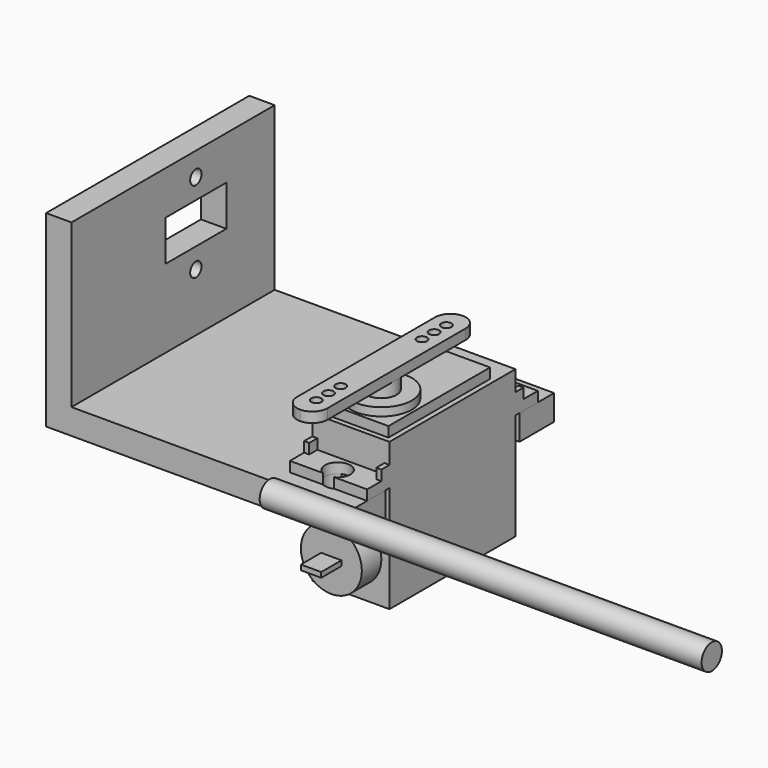
from build123d import *

# Parameters (mm, degrees)
F0_W      = 15.2
F0_H      = 31
F1_DEPTH  = 21
F3_DEPTH  = 2
F5_DEPTH  = 14.4
F4_W      = 1
F4_H      = 2
F6_DEPTH  = 2
F7_DEPTH  = 6
F8_R      = 6
F9_DEPTH  = 3.6
F8_W      = 13.2
F8_H      = 25
F10_DEPTH = 2
F11_R     = 3
F12_DEPTH = 2.6
F13_R     = 6
F14_DEPTH = 4.8
F15_W     = 4
F15_H     = 1
F16_DEPTH = 5
F18_DEPTH = 2
F19_R     = 1
F20_DEPTH = 2
F22_DEPTH = 5
F23_W     = 5
F23_H     = 50
F24_DEPTH = 32
F25_R     = 1.4
F25_W     = 15
F25_H     = 8
F26_DEPTH = 5
F27_R     = 2.7
F28_DEPTH = 2
F29_R     = 2.5
F30_DEPTH = 87


# Not quite as in the source:
# - an extrude ends at something that could not be found from the text; its depth is read off the source's solid


with BuildPart() as f1:
    # F0 (on Top) → F1 (new body)
    with BuildSketch(Plane.XY):
        with Locations((-7.6, 15.5)):
            Rectangle(F0_W, F0_H)
    extrude(amount=F1_DEPTH)

    # F2 (on face) → F3 (join)
    with BuildSketch(Plane.XY.offset(21)):
        Polygon((0, 36.5), (-15.2, 36.5), (-15.2, 31), (-15.2, 0), (-15.2, -5.5), (0, -5.5), (0, 0), (0, 31), align=None)
    extrude(amount=F3_DEPTH)

    # F4 (on face) → F5 (cut, through all)
    with BuildSketch(Plane.XY.offset(23)):
        with BuildLine():
            ThreePointArc((-6.5102752641, 36.5), (-7.6, 36.75), (-8.6897247359, 36.5))
            Line((-8.6897247359, 36.5), (-6.5102752641, 36.5))
        make_face()
        with BuildLine():
            Line((-6.5102752641, 36.5), (-8.6897247359, 36.5))
            ThreePointArc((-8.6897247359, 36.5), (-8.9277213865, 32.1317091985), (-5.1, 34.25))
            ThreePointArc((-5.1, 34.25), (-5.4817091985, 35.5777213865), (-6.5102752641, 36.5))
        make_face()
        with BuildLine():
            Line((-6.5102752641, -5.5), (-8.6897247359, -5.5))
            ThreePointArc((-8.6897247359, -5.5), (-7.6, -5.75), (-6.5102752641, -5.5))
        make_face()
        with BuildLine():
            ThreePointArc((-5.1, -3.25), (-8.9277213865, -1.1317091985), (-8.6897247359, -5.5))
            Line((-8.6897247359, -5.5), (-6.5102752641, -5.5))
            ThreePointArc((-6.5102752641, -5.5), (-5.4817091985, -4.5777213865), (-5.1, -3.25))
        make_face()
    extrude(amount=-F5_DEPTH, mode=Mode.SUBTRACT)

    # F4 (on face) → F6 (join)
    with BuildSketch(Plane.XY.offset(23)):
        with Locations((-14.7, 32)):
            Rectangle(F4_W, F4_H)
        with Locations((-0.5, 32)):
            Rectangle(F4_W, F4_H)
        with Locations((-0.5, -1)):
            Rectangle(F4_W, F4_H)
        with Locations((-14.7, -1)):
            Rectangle(F4_W, F4_H)
    extrude(amount=F6_DEPTH)

    # F4 (on face) → F7 (join)
    with BuildSketch(Plane.XY.offset(23)):
        Polygon((-14.2, 31), (-15.2, 31), (-15.2, 0), (-14.2, 0), (-1, 0), (0, 0), (0, 31), (-1, 31), align=None)
    extrude(amount=F7_DEPTH)

    # F8 (on face) → F9 (join)
    with BuildSketch(Plane.XY.offset(29)):
        with Locations((-7.6, 7.5)):
            Circle(F8_R)
    extrude(amount=F9_DEPTH)

    # F8 (on face) → F10 (join)
    with BuildSketch(Plane.XY.offset(29)):
        with Locations((-7.6, 13.5)):
            Rectangle(F8_W, F8_H)
        with Locations((-7.6, 7.5)):
            Circle(F8_R, mode=Mode.SUBTRACT)
    extrude(amount=F10_DEPTH)

    # F13 (on face) → F14 (join)
    with BuildSketch(Plane.XZ):
        with Locations((-7.6, 8.1)):
            Circle(F13_R)
    extrude(amount=F14_DEPTH)

    # F15 (on face) → F16 (join)
    with BuildSketch(Plane.XZ.offset(4.8)):
        with Locations((-7.6, 8.1)):
            Rectangle(F15_W, F15_H)
    extrude(amount=F16_DEPTH)


with BuildPart() as f12:
    # F11 (on face) → F12 (new body)
    with BuildSketch(Plane.XY.offset(32.6)):
        with Locations((-7.6, 7.5)):
            Circle(F11_R)
    extrude(amount=F12_DEPTH)

    # F17 (on face) → F18 (join)
    with BuildSketch(Plane.XY.offset(35.2)):
        with BuildLine():
            ThreePointArc((-7.6, 27.5), (-9.7213203436, 26.6213203436), (-10.6, 24.5))
            Line((-10.6, 24.5), (-10.6, -9.5))
            ThreePointArc((-10.6, -9.5), (-9.7213203436, -11.6213203436), (-7.6, -12.5))
            ThreePointArc((-7.6, -12.5), (-5.4786796564, -11.6213203436), (-4.6, -9.5))
            Line((-4.6, -9.5), (-4.6, 24.5))
            ThreePointArc((-4.6, 24.5), (-5.4786796564, 26.6213203436), (-7.6, 27.5))
        make_face()
    extrude(amount=F18_DEPTH)

    # F19 (on face) → F20 (cut, through all)
    with BuildSketch(Plane.XY.offset(37.2)):
        with Locations((-7.6, 23.5)):
            Circle(F19_R)
        with Locations((-7.6, -8.5)):
            Circle(F19_R)
        with Locations((-7.6, 20.5)):
            Circle(F19_R)
        with Locations((-7.6, 17.5)):
            Circle(F19_R)
        with Locations((-7.6, -2.5)):
            Circle(F19_R)
        with Locations((-7.6, -5.5)):
            Circle(F19_R)
    extrude(amount=-F20_DEPTH, mode=Mode.SUBTRACT)


with BuildPart() as f22:
    # F21 (on face) → F22 (new body)
    with BuildSketch(Plane(origin=(0, 0, 21), x_dir=(1, 0, 0), z_dir=(0, 0, -1))):
        with BuildLine():
            Line((0, 5.5), (0, 9.5))
            Line((0, 9.5), (-60, 9.5))
            Line((-60, 9.5), (-60, -40.5))
            Line((-60, -40.5), (0, -40.5))
            Line((0, -40.5), (0, -32))
            Line((0, -32), (-6.5102752641, -32))
            ThreePointArc((-6.5102752641, -32), (-5.4817091985, -32.9222786135), (-5.1, -34.25))
            ThreePointArc((-5.1, -34.25), (-8.9277213865, -36.3682908015), (-8.6897247359, -32))
            Line((-8.6897247359, -32), (-16, -32))
            Line((-16, -32), (-16, 1))
            Line((-16, 1), (-15.2, 1))
            Line((-15.2, 1), (-15.2, 5.5))
            Line((-15.2, 5.5), (-8.6897247359, 5.5))
            ThreePointArc((-8.6897247359, 5.5), (-7.6, 5.75), (-6.5102752641, 5.5))
            Line((-6.5102752641, 5.5), (0, 5.5))
        make_face()
        with BuildLine():
            Line((0, 1), (0, 5.5))
            Line((0, 5.5), (-6.5102752641, 5.5))
            ThreePointArc((-6.5102752641, 5.5), (-5.4817091985, 4.5777213865), (-5.1, 3.25))
            ThreePointArc((-5.1, 3.25), (-5.4817091985, 1.9222786135), (-6.5102752641, 1))
            Line((-6.5102752641, 1), (0, 1))
        make_face()
        with BuildLine():
            ThreePointArc((-8.6897247359, 1), (-10.1, 3.25), (-8.6897247359, 5.5))
            Line((-8.6897247359, 5.5), (-15.2, 5.5))
            Line((-15.2, 5.5), (-15.2, 1))
            Line((-15.2, 1), (-8.6897247359, 1))
        make_face()
    extrude(amount=F22_DEPTH)

    # F23 (on face) → F24 (join)
    with BuildSketch(Plane.XY.offset(21)):
        with Locations((-57.5, 15.5)):
            Rectangle(F23_W, F23_H)
    extrude(amount=F24_DEPTH)

    # F25 (on face) → F26 (cut, through all)
    with BuildSketch(Plane.YZ.offset(-55)):
        with Locations((21.1092480145, 48.4116717948)):
            Circle(F25_R)
        with Locations((21.1092480145, 32.4116717948)):
            Circle(F25_R)
        with Locations((21.1092480145, 40.4116717948)):
            Rectangle(F25_W, F25_H)
    extrude(amount=-F26_DEPTH, mode=Mode.SUBTRACT)

    # F27 (on face) → F28 (cut)
    with BuildSketch(Plane(origin=(-60, 0, 0), x_dir=(0, -1, 0), z_dir=(-1, 0, 0))):
        with Locations((-21.1092480145, 32.4116717948)):
            Circle(F27_R)
        with Locations((-21.1092480145, 48.4116717948)):
            Circle(F27_R)
    extrude(amount=-F28_DEPTH, mode=Mode.SUBTRACT)


with BuildPart() as f30:
    # F29 (on Right) → F30 (new body)
    with BuildSketch(Plane.YZ):
        with Locations((-29.4437985867, 32.0351906121)):
            Circle(F29_R)
    extrude(amount=F30_DEPTH)


solid = Compound([f1.part, f12.part, f22.part, f30.part])
